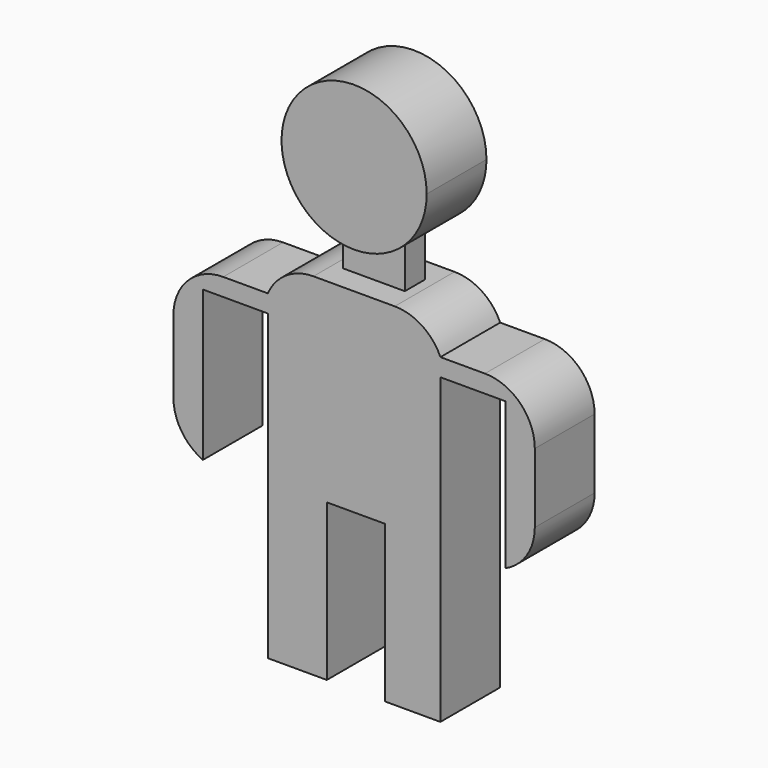
from build123d import *

# Parameters (mm, degrees)
F0_W        = 6.0157910921
F0_H        = 15.9466497103
F0_W_2      = 6.6173858
F0_H_2      = 1.8047373742
F0_W_3      = 6.6173737869
F0_W_4      = 5.6565788109
F0_W_5      = 6.2819751911
F0_H_3      = 2.8401233753
F1_DEPTH    = 3.81
F2_DEPTH    = 1.27
F3_R        = 5.08
F4_T1_DEPTH = 30.8109306563
F4_T3_DEPTH = 30.8109326237
F5_T1_DEPTH = 30.8932363866


# Not quite as in the source:
# - a fillet or chamfer that OpenCascade refuses, or shapes differently, is made with other operations: its cross-section is extruded or revolved along the edge and cut away or added


with BuildPart() as f1:
    # F0 (on Front) → F1 (new body, symmetric)
    with BuildSketch(Plane.XZ):
        Polygon((-3.1409875955, 26.922961697), (-3.1409875955, 29.7630850723), (-8.7975664064, 29.7630850723), (-8.7975664064, 26.7179459333), (-8.7975664064, 24.9132085592), (-8.7975664064, 9.9205921838), (-2.7817753144, 9.9205921838), (3.1409875955, 9.9205921838), (8.7975664064, 9.9205921838), (8.7975664064, 24.9132085592), (8.7975664064, 26.7179459333), (8.7975664064, 29.7630850723), (3.1409875955, 29.7630850723), (3.1409875955, 26.922961697), align=None)
        with Locations((-5.7896708604, 1.9472673287)):
            Rectangle(F0_W, F0_H)
        Polygon((-15.4149522064, 24.9132085592), (-15.4149522064, 26.7179459333), (-18.4228456064, 26.7179459333), (-18.4228456064, 9.6149956807), (-15.4149522064, 9.6149956807), align=None)
        with Locations((-12.1062593064, 25.8155772462)):
            Rectangle(F0_W_2, F0_H_2)
        Polygon((18.4228327125, 26.7179459333), (15.4149401933, 26.7179459333), (15.4149401933, 24.9132085592), (15.4149401933, 9.9205921838), (18.4228327125, 9.9205921838), align=None)
        with Locations((12.1062532999, 25.8155772462)):
            Rectangle(F0_W_3, F0_H_2)
        with Locations((5.969277001, 1.9472673287)):
            Rectangle(F0_W_4, F0_H)
        with Locations((0, 28.3430233846)):
            Rectangle(F0_W_5, F0_H_3)
    extrude(amount=F1_DEPTH, both=True)

    # F3
    f3_edges = [f1.edges().sort_by_distance(p)[0] for p in [
        (-18.422846, 0, 26.717946),
        (18.422833, 0, 26.717946),
    ]]
    fillet(f3_edges, radius=F3_R)

    # F4: fillet of radius 5.08 on 2 edges, made by hand

    # F4_s2 → F4_t1 (cut)
    with BuildSketch(Plane.XZ.offset(-15.4054653281)):
        with BuildLine():
            ThreePointArc((18.4228327125, 14.558778315), (17.6050332007, 11.794714821), (15.4149401933, 9.9205921838))
            Line((15.4149401933, 9.9205921838), (18.4228327125, 9.9205921838))
            Line((18.4228327125, 9.9205921838), (18.4228327125, 14.558778315))
        make_face()
    extrude(amount=F4_T1_DEPTH, mode=Mode.SUBTRACT)

    # F4_s4 → F4_t3 (cut)
    with BuildSketch(Plane.XZ.offset(-15.4054663118)):
        with BuildLine():
            ThreePointArc((-18.4228456064, 14.2531822055), (-17.6050458321, 11.4891183068), (-15.4149522064, 9.6149956807))
            Line((-15.4149522064, 9.6149956807), (-18.4228456064, 9.6149956807))
            Line((-18.4228456064, 9.6149956807), (-18.4228456064, 14.2531822055))
        make_face()
    extrude(amount=F4_T3_DEPTH, mode=Mode.SUBTRACT)

    # F5: fillet of radius 5.08 on 2 edges, made by hand

    # F5_s2 → F5_t1 (cut)
    with BuildSketch(Plane.XZ.offset(-15.4466181933)):
        with BuildLine():
            ThreePointArc((8.7975664064, 26.7179459333), (6.9240436163, 28.9341727669), (4.1429191291, 29.7630850723))
            Line((4.1429191291, 29.7630850723), (8.7975664064, 29.7630850723))
            Line((8.7975664064, 29.7630850723), (8.7975664064, 26.7179459333))
        make_face()
        with BuildLine():
            ThreePointArc((-8.7975664064, 26.7179459333), (-6.9240436163, 28.9341727669), (-4.1429191291, 29.7630850723))
            Line((-4.1429191291, 29.7630850723), (-8.7975664064, 29.7630850723))
            Line((-8.7975664064, 29.7630850723), (-8.7975664064, 26.7179459333))
        make_face()
    extrude(amount=F5_T1_DEPTH, mode=Mode.SUBTRACT)


with BuildPart() as f1b:
    # F0 (on Front) → F1, piece 2 (new body, symmetric)
    with BuildSketch(Plane.XZ):
        with BuildLine():
            ThreePointArc((3.1409875955, 34.2073870963), (6.2449143868, 36.9379106269), (7.3996991859, 40.9073680639))
            ThreePointArc((7.3996991859, 40.9073680639), (-3.969457437, 47.1522824507), (-3.1409875955, 34.2073870963))
            Line((-3.1409875955, 34.2073870963), (-3.1409875955, 40.092376059))
            Line((-3.1409875955, 40.092376059), (3.1409875955, 40.092376059))
            Line((3.1409875955, 40.092376059), (3.1409875955, 34.2073870963))
        make_face()
        with BuildLine():
            Line((-3.1409875955, 40.092376059), (-3.1409875955, 34.2073870963))
            ThreePointArc((-3.1409875955, 34.2073870963), (0, 33.507668878), (3.1409875955, 34.2073870963))
            Line((3.1409875955, 34.2073870963), (3.1409875955, 40.092376059))
            Line((3.1409875955, 40.092376059), (-3.1409875955, 40.092376059))
        make_face()
    extrude(amount=F1_DEPTH, both=True)


with BuildPart() as f2:
    # F0 (on Front) → F2 (new body, symmetric)
    with BuildSketch(Plane.XZ):
        with Locations((0, 28.3430233846)):
            Rectangle(F0_W_5, F0_H_3)
        with BuildLine():
            ThreePointArc((3.1409875955, 34.2073870963), (0, 33.507668878), (-3.1409875955, 34.2073870963))
            Line((-3.1409875955, 34.2073870963), (-3.1409875955, 29.7630850723))
            Line((-3.1409875955, 29.7630850723), (3.1409875955, 29.7630850723))
            Line((3.1409875955, 29.7630850723), (3.1409875955, 34.2073870963))
        make_face()
        with BuildLine():
            Line((-3.1409875955, 40.092376059), (-3.1409875955, 34.2073870963))
            ThreePointArc((-3.1409875955, 34.2073870963), (0, 33.507668878), (3.1409875955, 34.2073870963))
            Line((3.1409875955, 34.2073870963), (3.1409875955, 40.092376059))
            Line((3.1409875955, 40.092376059), (-3.1409875955, 40.092376059))
        make_face()
    extrude(amount=F2_DEPTH, both=True)


solid = Compound([f1.part, f1b.part, f2.part])
